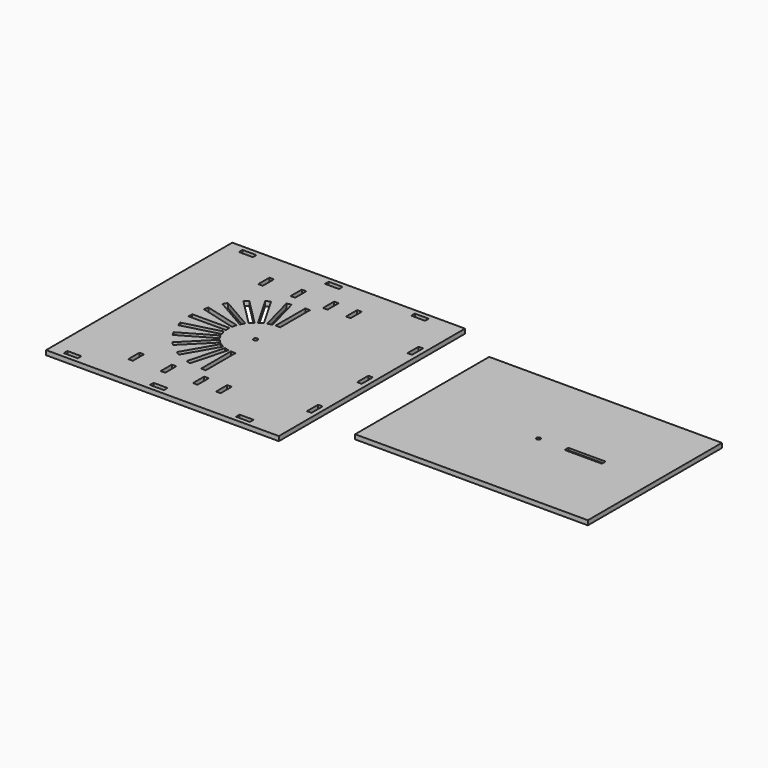
from build123d import *

# Parameters (mm, degrees)
F0_W     = 635
F0_H     = 635
F0_R     = 5.55625
F1_DEPTH = 12.3952
F0_H_2   = 457.2
F0_W_2   = 101.6
F0_H_3   = 12.7
F2_W     = 38.1
F2_H     = 12.3952
F2_W_2   = 12.3952
F2_H_2   = 38.1
F2_H_3   = 19.05
F3_DEPTH = 12.3952
F4_DEPTH = 6.35
F5_W     = 12.7
F5_H     = 101.6
F5_W_2   = 101.6
F5_H_2   = 12.7
F6_DEPTH = 12.3952


# Not quite as in the source:
# - a feature names something its author has since deleted; it is built from what else it names


with BuildPart() as f1:
    # F0 (on Top) → F1 (new body)
    with BuildSketch(Plane.XY):
        with Locations((317.5, 317.5)):
            Rectangle(F0_W, F0_H)
        with Locations((317.5, 317.5)):
            Circle(F0_R, mode=Mode.SUBTRACT)
    extrude(amount=F1_DEPTH)

    # F2 (on face) → F3 (cut)
    with BuildSketch(Plane.XY.offset(12.3952)):
        with Locations((57.15, 616.1024)):
            Rectangle(F2_W, F2_H)
        with Locations((292.1, 616.1024)):
            Rectangle(F2_W, F2_H)
        with Locations((527.05, 616.1024)):
            Rectangle(F2_W, F2_H)
        with Locations((57.15, 18.8976)):
            Rectangle(F2_W, F2_H)
        with Locations((292.1, 18.8976)):
            Rectangle(F2_W, F2_H)
        with Locations((527.05, 18.8976)):
            Rectangle(F2_W, F2_H)
        with Locations((616.1024, 488.95)):
            Rectangle(F2_W_2, F2_H_2)
        with Locations((616.1024, 327.025)):
            Rectangle(F2_W_2, F2_H_3)
        with Locations((616.1024, 146.05)):
            Rectangle(F2_W_2, F2_H_2)
        with Locations((408.399107, 95.8469)):
            Rectangle(F2_W_2, F2_H_2)
        with Locations((345.508707, 95.8342)):
            Rectangle(F2_W_2, F2_H_2)
        with Locations((168.927907, 95.8342)):
            Rectangle(F2_W_2, F2_H_2)
        with Locations((257.218307, 95.8342)):
            Rectangle(F2_W_2, F2_H_2)
        with Locations((168.927907, 539.1522364)):
            Rectangle(F2_W_2, F2_H_2)
        with Locations((257.218307, 539.1522364)):
            Rectangle(F2_W_2, F2_H_2)
        with Locations((345.508707, 539.1522364)):
            Rectangle(F2_W_2, F2_H_2)
        with Locations((408.399107, 539.1522364)):
            Rectangle(F2_W_2, F2_H_2)
        with Locations((616.1024, 307.975)):
            Rectangle(F2_W_2, F2_H_3)
    extrude(amount=-F3_DEPTH, mode=Mode.SUBTRACT)

    # F5 (on face) → F6 (cut, through all)
    with BuildSketch(Plane.XY.offset(12.3952)):
        with Locations((317.5, 444.5)):
            Rectangle(F5_W, F5_H)
        Polygon((303.9116177601, 392.7470488996), (277.6156027777, 490.8851128506), (265.3483447838, 487.5981109778), (291.6443597663, 389.4600470268), align=None)
        Polygon((284.899261314, 386.6661357684), (234.099261314, 474.6543167929), (223.100738686, 468.3043167929), (273.900738686, 380.3161357684), align=None)
        Polygon((259.1283352131, 366.8914086659), (268.1085913341, 375.8716647869), (196.2665423656, 447.7137137555), (187.2862862445, 438.7334576344), align=None)
        Polygon((248.3338642316, 350.100738686), (254.6838642316, 361.099261314), (166.6956832071, 411.899261314), (160.3456832071, 400.900738686), align=None)
        Polygon((242.2529511004, 331.0883822399), (245.5399529732, 343.3556402337), (147.4018890222, 369.6516552162), (144.1148871494, 357.3843972223), align=None)
        with Locations((190.5, 317.5)):
            Rectangle(F5_W_2, F5_H_2)
        Polygon((245.5399529732, 291.6443597663), (242.2529511004, 303.9116177601), (144.1148871494, 277.6156027777), (147.4018890222, 265.3483447838), align=None)
        Polygon((254.6838642316, 273.900738686), (248.3338642316, 284.899261314), (160.3456832071, 234.099261314), (166.6956832071, 223.100738686), align=None)
        Polygon((268.1085913341, 259.1283352131), (259.1283352131, 268.1085913341), (187.2862862445, 196.2665423656), (196.2665423656, 187.2862862445), align=None)
        Polygon((284.899261314, 248.3338642316), (273.900738686, 254.6838642316), (223.100738686, 166.6956832071), (234.099261314, 160.3456832071), align=None)
        Polygon((303.9116177601, 242.2529511004), (291.6443597663, 245.5399529732), (265.3483447838, 147.4018890222), (277.6156027777, 144.1148871494), align=None)
        with Locations((317.5, 190.5)):
            Rectangle(F5_W, F5_H)
    extrude(amount=-F6_DEPTH, mode=Mode.SUBTRACT)


with BuildPart() as f1b:
    # F0 (on Top) → F1, piece 2 (new body)
    with BuildSketch(Plane.XY):
        with Locations((1074.0928434372, 336.6985905102)):
            Rectangle(F0_W, F0_H_2)
        with Locations((1074.0928434372, 336.6985905102)):
            Circle(F0_R, mode=Mode.SUBTRACT)
        with Locations((1201.0928434372, 336.6985905102)):
            Rectangle(F0_W_2, F0_H_3, mode=Mode.SUBTRACT)
    extrude(amount=F1_DEPTH)

    # F0 (on Top) → F4 (join)
    with BuildSketch(Plane.XY):
        with Locations((1201.0928434372, 336.6985905102)):
            Rectangle(F0_W_2, F0_H_3)
    extrude(amount=F4_DEPTH)


solid = Compound([f1.part, f1b.part])
